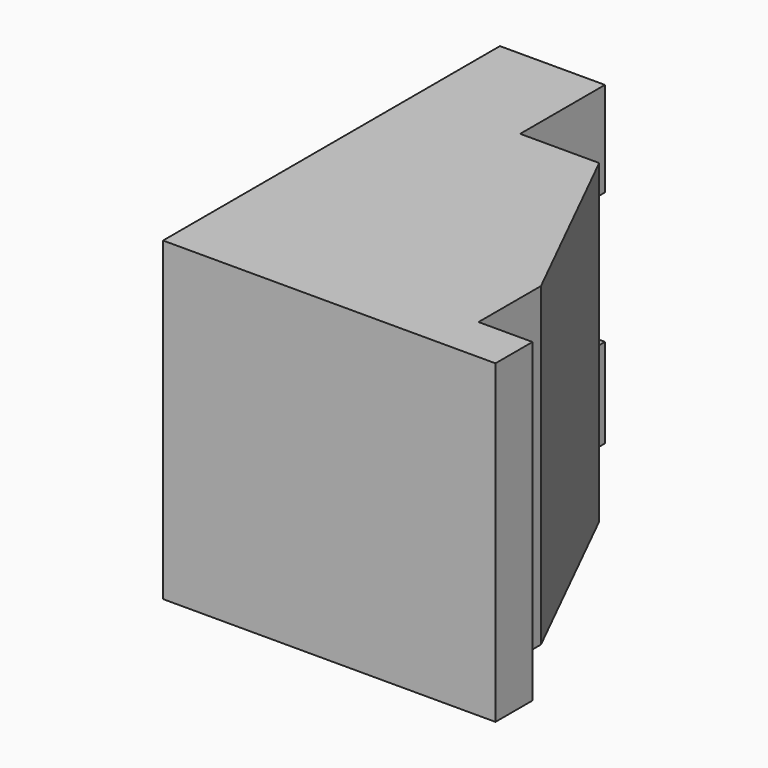
from build123d import *

# Parameters (mm, degrees)
F0_W      = 89.0809036791
F0_H      = 101.640611887
F1_DEPTH  = 76.2
F3_DEPTH  = 76.201
F4_R      = 10.6888946351
F3_FACE_W = 51.3844064591
F3_FACE_H = 76.2
F5_DEPTH  = 12.7
F8_W      = 6.35
F8_H      = 31.75
F9_DEPTH  = 25.4


# Not quite as in the source:
# - a feature of the source that left no trace in its solid (it failed there, or was rolled back) is left out


with BuildPart() as f1:
    # F0 (on Top) → F1 (new body)
    with BuildSketch(Plane.XY):
        with Locations((-6.628734991, 2.674754709)):
            Rectangle(F0_W, F0_H)
    extrude(amount=F1_DEPTH)

    # F2 (on face) → F3 (cut, through all)
    with BuildSketch(Plane.XY.offset(76.2)):
        Polygon((37.9117168486, 53.4950606525), (-25.8171800524, 53.4950606525), (-25.8171800524, 27.9104653746), (-6.7450297065, 27.9104653746), (16.0485189408, -18.1418024004), (16.0485189408, -36.9813665748), (29.0734022856, -36.9813665748), (29.0734022856, -48.1455512345), (31.1666838825, -48.1455512345), (37.9117168486, -48.1455512345), align=None)
    extrude(amount=-F3_DEPTH, mode=Mode.SUBTRACT)

    # F4 (on Right) + F3_face (on face) → F5 (join)
    with BuildSketch(Plane.YZ):
        with Locations((0, 59.542324394)):
            Circle(F4_R)
    with BuildSketch(Plane(origin=(4.6517446171, 4.8843314871, 38.1), x_dir=(-0.4435888282, 0.8962304121, 0), z_dir=(0.8962304121, 0.4435888282, 0))):
        Rectangle(F3_FACE_W, F3_FACE_H)
    extrude(amount=-F5_DEPTH, dir=(1, 0, 0))

    # F8 (on face) → F9 (cut)
    with BuildSketch(Plane(origin=(0, 53.4950606525, 0), x_dir=(-1, 0, 0), z_dir=(0, 1, 0))):
        with Locations((28.9921800524, 37.465)):
            Rectangle(F8_W, F8_H)
    extrude(amount=-F9_DEPTH, mode=Mode.SUBTRACT)


solid = f1.part
